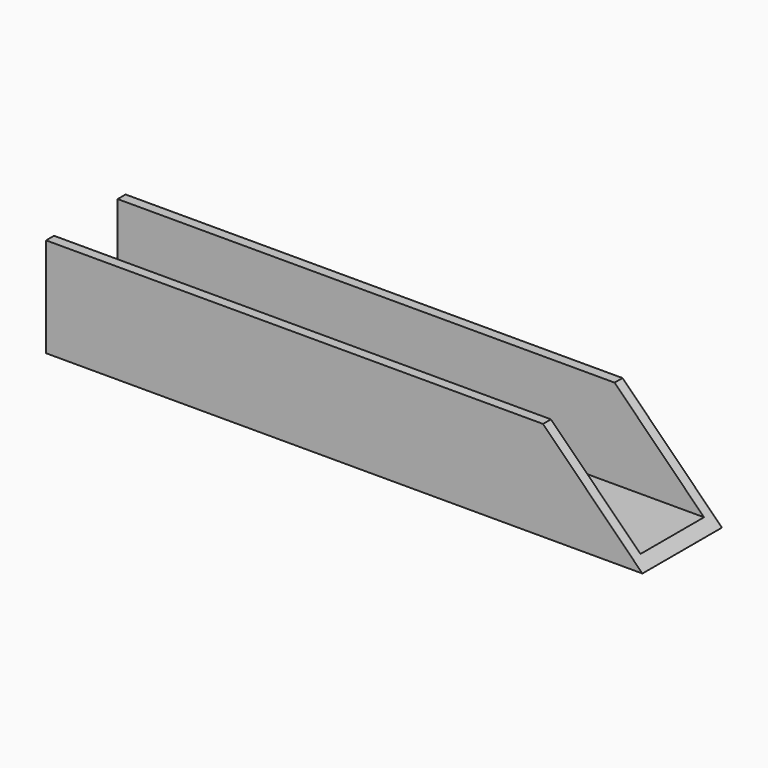
from build123d import *

# Parameters (mm, degrees)
F1_DEPTH   = 60
F2_C1_SIZE = 9.9999


# Not quite as in the source:
# - a fillet or chamfer is up to 0.001 mm smaller than in the source, because OpenCascade refuses the exact size


with BuildPart() as f1:
    # F0 (on Right) → F1 (new body)
    with BuildSketch(Plane.YZ):
        Polygon((-4, 5), (-5, 5), (-5, -5), (5, -5), (5, 5), (4, 5), (4, -4), (-4, -4), align=None)
    extrude(amount=F1_DEPTH)

    # F2: chamfer of 10 on 2 edges, made by hand

    # F2_c1 (size 10 in the source; OpenCascade refuses exactly that, so slightly less here)
    f2_c1_edges = [f1.edges().sort_by_distance(p)[0] for p in [
        (60, -4.5, 5),
    ]]
    chamfer(f2_c1_edges, length=F2_C1_SIZE)


solid = f1.part
